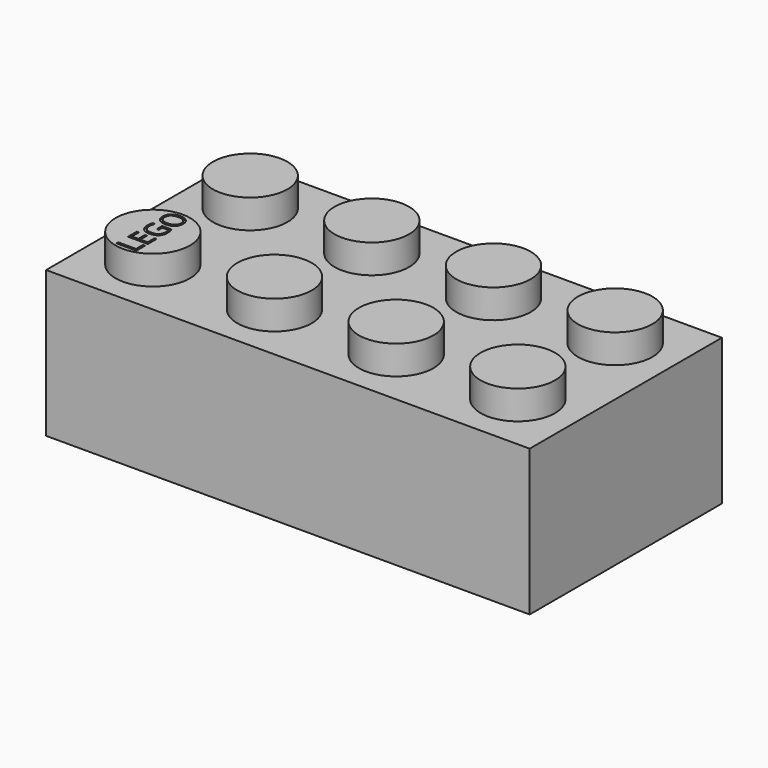
from build123d import *

# Parameters (mm, degrees)
F0_W         = 31.8
F0_H         = 15.8
F1_DEPTH     = 9.6
F2_R         = 2.45
F3_DEPTH     = 1.9
F4_R         = 3.205
F4_R_2       = 2.45
F5_DEPTH     = 7
F6_TEXT_SIZE = 1.8255309229
F7_DEPTH     = 0.1


# Not quite as in the source:
# - Text() gives the source's letters only with a copy of the font that has no kerning and outlines rounded to 1/6400 em; it was checked with that copy


with BuildPart() as f1:
    # F0 (on Top) → F1 (new body)
    with BuildSketch(Plane.XY):
        with Locations((15.9, 7.9)):
            Rectangle(F0_W, F0_H)
    extrude(amount=F1_DEPTH)

    # F2 (on face) → F3 (join)
    with BuildSketch(Plane.XY.offset(9.6)):
        with Locations((3.9, 3.9)):
            Circle(F2_R)
        with Locations((3.9, 11.9)):
            Circle(F2_R)
        with Locations((11.9, 3.9)):
            Circle(F2_R)
        with Locations((11.9, 11.9)):
            Circle(F2_R)
        with Locations((19.9, 3.9)):
            Circle(F2_R)
        with Locations((19.9, 11.9)):
            Circle(F2_R)
        with Locations((27.9, 3.9)):
            Circle(F2_R)
        with Locations((27.9, 11.9)):
            Circle(F2_R)
    extrude(amount=F3_DEPTH)

    # F4 (on face) → F5 (cut)
    with BuildSketch(Plane(origin=(0, 0, 0), x_dir=(1, 0, 0), z_dir=(0, 0, -1))):
        Polygon((30.6315632832, -3.6), (30.6315632832, -1.1684367168), (28.2, -1.1684367168), (28.2, -1.4684367168), (27.6, -1.4684367168), (27.6, -1.1684367168), (20.2, -1.1684367168), (20.2, -1.4684367168), (19.6, -1.4684367168), (19.6, -1.1684367168), (12.2, -1.1684367168), (12.2, -1.4684367168), (11.6, -1.4684367168), (11.6, -1.1684367168), (4.2, -1.1684367168), (4.2, -1.4684367168), (3.6, -1.4684367168), (3.6, -1.1684367168), (1.1684367168, -1.1684367168), (1.1684367168, -3.6), (1.4684367168, -3.6), (1.4684367168, -4.2), (1.1684367168, -4.2), (1.1684367168, -11.6), (1.4684367168, -11.6), (1.4684367168, -12.2), (1.1684367168, -12.2), (1.1684367168, -14.6315632832), (3.6, -14.6315632832), (3.6, -14.3315632832), (4.2, -14.3315632832), (4.2, -14.6315632832), (11.6, -14.6315632832), (11.6, -14.3315632832), (12.2, -14.3315632832), (12.2, -14.6315632832), (19.6, -14.6315632832), (19.6, -14.3315632832), (20.2, -14.3315632832), (20.2, -14.6315632832), (27.6, -14.6315632832), (27.6, -14.3315632832), (28.2, -14.3315632832), (28.2, -14.6315632832), (30.6315632832, -14.6315632832), (30.6315632832, -12.2), (30.3315632832, -12.2), (30.3315632832, -11.6), (30.6315632832, -11.6), (30.6315632832, -4.2), (30.3315632832, -4.2), (30.3315632832, -3.6), align=None)
        with Locations((7.9, -7.9)):
            Circle(F4_R, mode=Mode.SUBTRACT)
        with Locations((15.9, -7.9)):
            Circle(F4_R, mode=Mode.SUBTRACT)
        with Locations((23.9, -7.9)):
            Circle(F4_R, mode=Mode.SUBTRACT)
        with Locations((7.9, -7.9)):
            Circle(F4_R_2)
        with Locations((15.9, -7.9)):
            Circle(F4_R_2)
        with Locations((23.9, -7.9)):
            Circle(F4_R_2)
    extrude(amount=-F5_DEPTH, mode=Mode.SUBTRACT)

    # F6 (on face) → F7 (cut)
    with BuildSketch(Plane.XY.offset(11.5)):
        with Locations(Location((4.5571911322, 1.5397881841), (0, 0, 90))):
            Text('LEGO', F6_TEXT_SIZE, font='Open Sans', text_align=(TextAlign.LEFT, TextAlign.BOTTOM))
    extrude(amount=-F7_DEPTH, mode=Mode.SUBTRACT)


solid = f1.part
